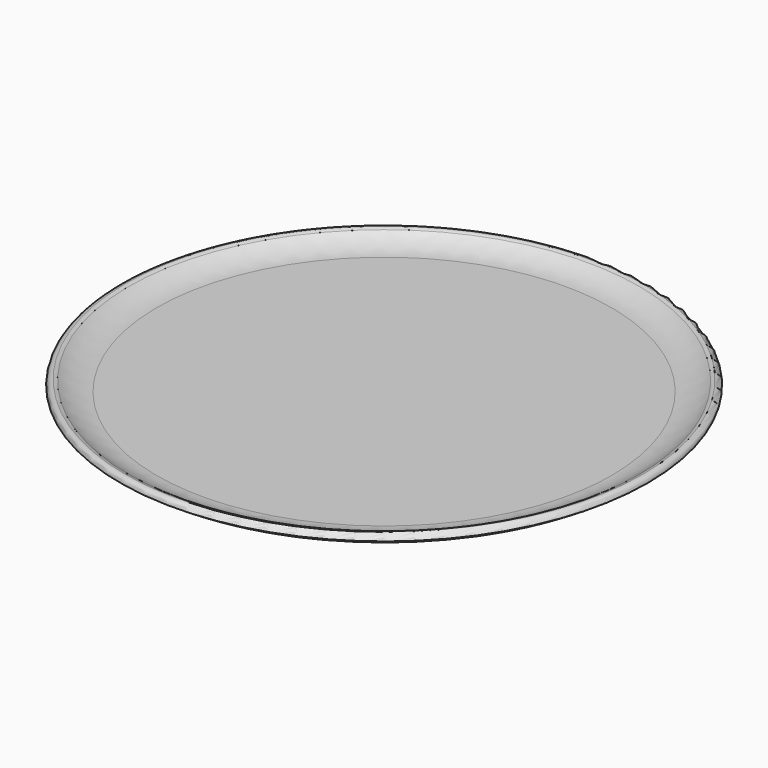
from build123d import *

# Parameters (mm, degrees)
F0_R     = 76.2
F1_DEPTH = 6.35
F2_R     = 73.025
F3_DEPTH = 3.175
F5_R     = 12.7


# Not quite as in the source:
# - a fillet or chamfer that OpenCascade refuses, or shapes differently, is made with other operations: its cross-section is extruded or revolved along the edge and cut away or added


with BuildPart() as f1:
    # F0 (on Top) → F1 (new body)
    with BuildSketch(Plane.XY):
        Circle(F0_R)
    extrude(amount=F1_DEPTH)

    # F2 (on face) → F3 (cut)
    with BuildSketch(Plane.XY.offset(6.35)):
        Circle(F2_R)
    extrude(amount=-F3_DEPTH, mode=Mode.SUBTRACT)

    # F4: fillet of radius 1.5875 on 2 edges, made by hand

    # F4_s1 → F4_t2 (revolve, cut)
    with BuildSketch(Plane.XZ):
        with BuildLine():
            ThreePointArc((74.6125, 6.35), (73.4899679849, 5.8850320151), (73.025, 4.7625))
            Line((73.025, 4.7625), (73.025, 6.35))
            Line((73.025, 6.35), (74.6125, 6.35))
        make_face()
    revolve(axis=Axis((0, 0, 6.35), (0, 0, 1)), mode=Mode.SUBTRACT)

    # F4_s3 → F4_t4 (revolve, cut)
    with BuildSketch(Plane.XZ):
        with BuildLine():
            ThreePointArc((76.2, 4.7625), (75.7350320151, 5.8850320151), (74.6125, 6.35))
            Line((74.6125, 6.35), (76.2, 6.35))
            Line((76.2, 6.35), (76.2, 4.7625))
        make_face()
    revolve(axis=Axis((0, 0, 6.35), (0, 0, 1)), mode=Mode.SUBTRACT)

    # F5
    f5_edges = [f1.edges().sort_by_distance(p)[0] for p in [
        (-73.025, 0, 3.175),
    ]]
    fillet(f5_edges, radius=F5_R)

    # F6: fillet of radius 25.4 on 1 edges, made by hand

    # F6_s1 → F6_t2 (revolve, cut)
    with BuildSketch(Plane.XZ):
        with BuildLine():
            ThreePointArc((76.2, 4.7625), (69.1699156866, 1.2199203889), (61.3927857532, 0))
            Line((61.3927857532, 0), (61.3927857532, -0.508))
            Line((61.3927857532, -0.508), (76.2, -0.508))
            Line((76.2, -0.508), (76.708, 0))
            ThreePointArc((76.708, 0), (76.708, 2.38125), (76.4961442849, 4.34975))
            Line((76.4961442849, 4.34975), (76.2, 4.7625))
        make_face()
    revolve(axis=Axis((0, 0, 0), (0, 0, 1)), mode=Mode.SUBTRACT)


solid = f1.part
